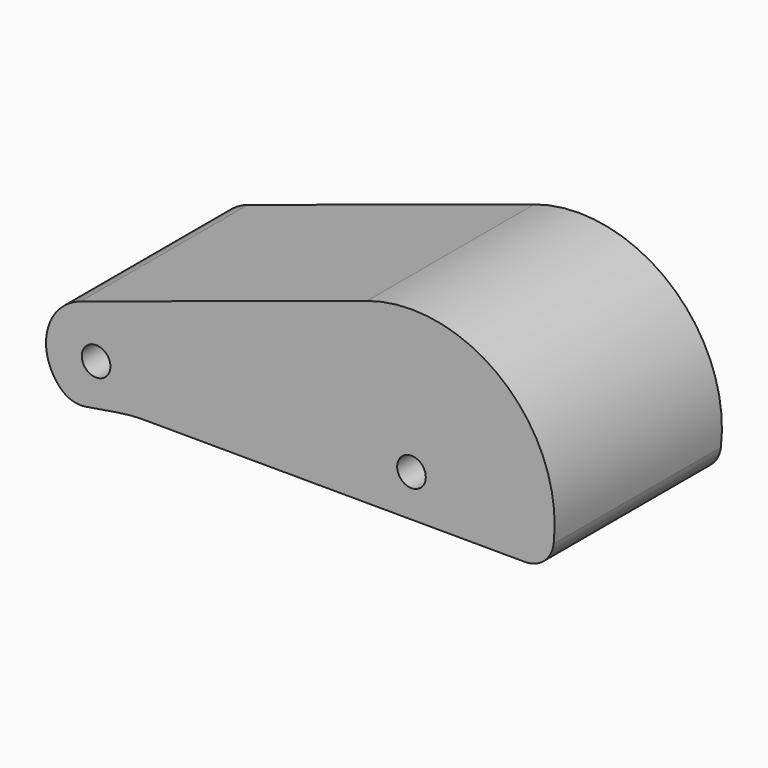
from build123d import *

# Parameters (mm, degrees)
F0_R        = 5
F1_DEPTH    = 73
F2_T1_DEPTH = 73
F3_R        = 10
F4_T        = 2.5


# Not quite as in the source:
# - a fillet or chamfer that OpenCascade refuses, or shapes differently, is made with other operations: its cross-section is extruded or revolved along the edge and cut away or added
# - a shell that OpenCascade refuses in one call is made with other operations: the cavity is built on its own and cut out


with BuildPart() as f1:
    # F0 (on Front) → F1 (new body)
    with BuildSketch(Plane.XZ):
        with BuildLine():
            Line((105.4664104798, -2.1604888337), (110.723299262, -2.1771916507))
            ThreePointArc((110.723299262, -2.1771916507), (98.0443002081, 48.2472921113), (47.4300209604, 60.1460448152))
            Line((47.4300209604, 60.1460448152), (-52.5831548864, 27.4585928761))
            ThreePointArc((-52.5831548864, 27.4585928761), (-64.6091493054, 11.9687796957), (-54.7073812284, -4.9579401011))
            Line((-54.7073812284, -4.9579401011), (-34.93893119, -1.7143761565))
            Line((-34.93893119, -1.7143761565), (20.3665836392, -1.8900994658))
            ThreePointArc((20.3665836392, -1.8900994658), (55.6091219512, 57.015037844), (107.9630298197, 12.6199926356))
            ThreePointArc((107.9630298197, 12.6199926356), (107.3344853384, 5.1250653412), (105.4664104798, -2.1604888337))
        make_face()
        with Locations((-47.1466017857, 10.8244746133)):
            Circle(F0_R, mode=Mode.SUBTRACT)
        with BuildLine():
            Line((20.3665836392, -1.8900994658), (105.4664104798, -2.1604888337))
            ThreePointArc((105.4664104798, -2.1604888337), (107.3344853384, 5.1250653412), (107.9630298197, 12.6199926356))
            ThreePointArc((107.9630298197, 12.6199926356), (55.6091219512, 57.015037844), (20.3665836392, -1.8900994658))
        make_face()
        with Locations((62.9630298197, 12.6199926356)):
            Circle(F0_R, mode=Mode.SUBTRACT)
    extrude(amount=F1_DEPTH)

    # F2: fillet of radius 60 on 1 edges, made by hand

    # F2_s2 → F2_t1 (join)
    with BuildSketch(Plane.XZ):
        with BuildLine():
            add(Edge.make_bspline(
                [(-39.8587548674, -2.52161004), (-34.93893119, -1.7143761565), (-29.9533479112, -1.7302169492)],
                knots=[0, 0, 0, 1, 1, 1], degree=2, weights=[1, 1, 1]))
            Line((-29.9533479112, -1.7302169492), (-34.93893119, -1.7143761565))
            Line((-34.93893119, -1.7143761565), (-39.8587548674, -2.52161004))
        make_face()
    extrude(amount=F2_T1_DEPTH)

    # F3
    f3_edges = [f1.edges().sort_by_distance(p)[0] for p in [
        (110.723299, -36.5, -2.177192),
        (-54.707381, -36.5, -4.95794),
    ]]
    fillet(f3_edges, radius=F3_R)

    # F4: shell of thickness 2.5, made by hand


with BuildPart() as f4_core1:
    # F4_t2: copy of F1
    add(f1.part)

    # the walls: a layer under each face that stays
    f4_faces = [f4_core1.faces().sort_by_distance(p)[0] for p in [
        (94.683390136, -36.5, 51.2699440121),
        (24.158214017, 0, 29.0813282585),
        (109.3014464934, -36.5, 0.3569505301),
        (-2.576566963, -36.5, 43.8023188457),
        (24.158214017, -73, 29.0813282585),
        (-64.1583335829, -36.5, 14.9294692855),
        (-55.554318165, -36.5, -3.9702240205),
        (-45.3554663929, -36.5, -3.4234984168),
        (-52.1466017857, -36.5, 10.8244746133),
        (57.9630298197, -36.5, 12.6199926356),
    ]]
    thicken(f4_faces, amount=-F4_T, mode=Mode.SUBTRACT)


with BuildPart() as f1_1:
    add(f1.part)

    # what is left inside the walls is the cavity
    f4_cavity = [f4_core1.part.solids().sort_by_distance(p)[0] for p in [
        (36.346225, -47.833333, -1.915872),
    ]]
    add(f4_cavity, mode=Mode.SUBTRACT)


solid = f1_1.part
